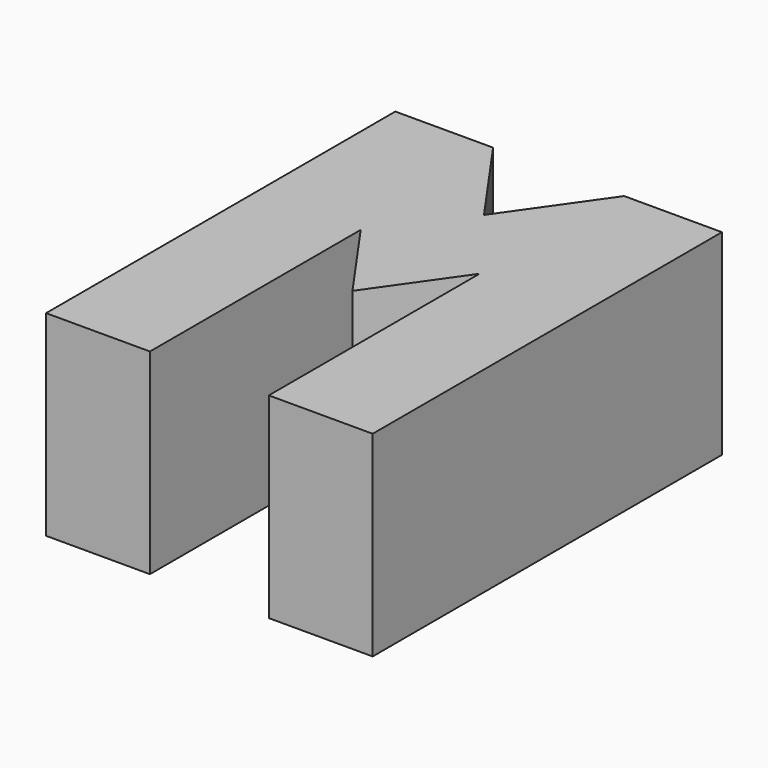
from build123d import *

# Parameters (mm, degrees)
F0_W          = 29.8302113987
F0_H          = 9.2097856104
F1_DEPTH      = 25.4
F2_T1_DEPTH   = 25.4
F2_T3_DEPTH   = 15.24
F2_T5_DEPTH   = 56.4671399768
F2_T7_DEPTH   = 44.9504289544
F2_T9_DEPTH   = 56.4670330548
F2_T11_DEPTH  = 20.32
F2_T13_DEPTH  = 20.3101045111
F2_T15_DEPTH  = 50.8
F2_T20_DEPTH  = 5.08
F2_T26_DEPTH  = 5.08
F2_T32_DEPTH  = 5.08
F2_T38_DEPTH  = 5.08
F2_S43_W      = 5.08
F2_S43_H      = 5.08
F2_T44_DEPTH  = 5.08
F2_S49_W      = 5.08
F2_S49_H      = 5.08
F2_T50_DEPTH  = 5.08
F2_S55_W      = 5.08
F2_S55_H      = 5.08
F2_T56_DEPTH  = 5.08
F2_S61_W      = 5.08
F2_S61_H      = 5.08
F2_T62_DEPTH  = 5.08
F2_T65_DEPTH  = 11.1376243347
F2_T67_DEPTH  = 11.5693333262
F2_T69_DEPTH  = 19.6702113987
F2_S73_W      = 5.08
F2_S73_H      = 5.08
F2_T74_DEPTH  = 5.08
F2_S79_W      = 5.08
F2_S79_H      = 5.08
F2_T80_DEPTH  = 5.08
F2_S85_W      = 5.08
F2_S85_H      = 5.08
F2_T86_DEPTH  = 5.08
F2_S91_W      = 5.08
F2_S91_H      = 5.08
F2_T92_DEPTH  = 5.08
F2_T96_ANGLE  = 90
F2_T98_ANGLE  = 90
F2_T100_ANGLE = 90
F2_T102_ANGLE = 90
F2_T104_ANGLE = 90
F2_T106_ANGLE = 90
F2_T108_ANGLE = 90
F2_T110_ANGLE = 90
F2_T112_ANGLE = 90
F2_T114_ANGLE = 90
F2_T116_ANGLE = 90
F2_T118_ANGLE = 90
F3_DEPTH      = 25.4
F6_DEPTH      = 25.4


# Not quite as in the source:
# - a fillet or chamfer that OpenCascade refuses, or shapes differently, is made with other operations: its cross-section is extruded or revolved along the edge and cut away or added


with BuildPart() as f1:
    # F0 (on Top) → F1 (new body)
    with BuildSketch(Plane.XY):
        Polygon((-27.6151056993, 52.1290511863), (-27.6151056993, 0), (-14.9151056993, 0), (-14.9151056993, 21.7293333262), (-14.9151056993, 30.9391189367), (-14.9151056993, 52.2367432714), (14.9151056993, 52.2367432714), (14.9151056993, 30.9391189367), (14.9151056993, 21.7293333262), (14.9151056993, 0), (27.6151056993, 0), (27.4854470044, 66.6270330548), (-27.6151056993, 66.6270330548), align=None)
        with Locations((0, 26.3342261314)):
            Rectangle(F0_W, F0_H)
    extrude(amount=F1_DEPTH)

    # F2: fillet of radius 5.08 on 36 edges, made by hand

    # F2_s2 → F2_t1 (join)
    with BuildSketch(Plane.XY):
        with BuildLine():
            ThreePointArc((-14.9151056993, 36.0191189367), (-13.4272081478, 32.4270164882), (-9.8351056993, 30.9391189367))
            Line((-9.8351056993, 30.9391189367), (-14.9151056993, 30.9391189367))
            Line((-14.9151056993, 30.9391189367), (-14.9151056993, 36.0191189367))
        make_face()
        with BuildLine():
            ThreePointArc((-14.9151056993, 47.1567432714), (-13.4272081478, 50.7488457198), (-9.8351056993, 52.2367432714))
            Line((-9.8351056993, 52.2367432714), (-14.9151056993, 52.2367432714))
            Line((-14.9151056993, 52.2367432714), (-14.9151056993, 47.1567432714))
        make_face()
        with BuildLine():
            ThreePointArc((9.8351056993, 52.2367432714), (13.4272081478, 50.7488457198), (14.9151056993, 47.1567432714))
            Line((14.9151056993, 47.1567432714), (14.9151056993, 52.2367432714))
            Line((14.9151056993, 52.2367432714), (9.8351056993, 52.2367432714))
        make_face()
        with BuildLine():
            ThreePointArc((14.9151056993, 36.0191189367), (13.4272081478, 32.4270164882), (9.8351056993, 30.9391189367))
            Line((9.8351056993, 30.9391189367), (14.9151056993, 30.9391189367))
            Line((14.9151056993, 30.9391189367), (14.9151056993, 36.0191189367))
        make_face()
        with BuildLine():
            ThreePointArc((9.8351056993, 21.7293333262), (13.4272081478, 20.2414357746), (14.9151056993, 16.6493333262))
            Line((14.9151056993, 16.6493333262), (14.9151056993, 21.7293333262))
            Line((14.9151056993, 21.7293333262), (9.8351056993, 21.7293333262))
        make_face()
        with BuildLine():
            ThreePointArc((-14.9151056993, 16.6493333262), (-13.4272081478, 20.2414357746), (-9.8351056993, 21.7293333262))
            Line((-9.8351056993, 21.7293333262), (-14.9151056993, 21.7293333262))
            Line((-14.9151056993, 21.7293333262), (-14.9151056993, 16.6493333262))
        make_face()
    extrude(amount=F2_T1_DEPTH)

    # F2_s4 → F2_t3 (cut)
    with BuildSketch(Plane.XY.offset(5.08)):
        with BuildLine():
            ThreePointArc((27.6052005914, 5.089885851), (26.1208061363, 1.4913944298), (22.5252102105, 0))
            Line((22.5252102105, 0), (27.6151056993, 0))
            Line((27.6151056993, 0), (27.6052005914, 5.089885851))
        make_face()
        with BuildLine():
            ThreePointArc((22.4153232551, 66.6270330548), (26.0039288252, 65.1426289806), (27.4953136359, 61.5569189059))
            Line((27.4953136359, 61.5569189059), (27.4854470044, 66.6270330548))
            Line((27.4854470044, 66.6270330548), (22.4153232551, 66.6270330548))
        make_face()
        with BuildLine():
            ThreePointArc((-22.5351056993, 66.6270330548), (-26.1272081478, 65.1391355033), (-27.6151056993, 61.5470330548))
            Line((-27.6151056993, 61.5470330548), (-27.6151056993, 66.6270330548))
            Line((-27.6151056993, 66.6270330548), (-22.5351056993, 66.6270330548))
        make_face()
        with BuildLine():
            ThreePointArc((-27.6151056993, 5.08), (-26.1272081478, 1.4878975516), (-22.5351056993, 0))
            Line((-22.5351056993, 0), (-27.6151056993, 0))
            Line((-27.6151056993, 0), (-27.6151056993, 5.08))
        make_face()
    extrude(amount=F2_T3_DEPTH, mode=Mode.SUBTRACT)

    # F2_s6 → F2_t5 (cut)
    with BuildSketch(Plane(origin=(-0.0098005283, 5.0361460274, 0), x_dir=(0, 0, 1), z_dir=(-0.0019460337, 0.9999981065, 0))):
        with BuildLine():
            ThreePointArc((5.08, 27.6150534094), (1.4878975516, 26.1271558579), (0, 22.5350534094))
            Line((0, 22.5350534094), (0, 27.6150534094))
            Line((0, 27.6150534094), (5.08, 27.6150534094))
        make_face()
        with BuildLine():
            ThreePointArc((20.32, 27.6150534094), (23.9121024484, 26.1271558579), (25.4, 22.5350534094))
            Line((25.4, 22.5350534094), (25.4, 27.6150534094))
            Line((25.4, 27.6150534094), (20.32, 27.6150534094))
        make_face()
    extrude(amount=F2_T5_DEPTH, mode=Mode.SUBTRACT)

    # F2_s8 → F2_t7 (cut)
    with BuildSketch(Plane.YZ.offset(-22.5351056993)):
        with BuildLine():
            ThreePointArc((66.6270330548, 5.08), (65.1391355033, 1.4878975516), (61.5470330548, 0))
            Line((61.5470330548, 0), (66.6270330548, 0))
            Line((66.6270330548, 0), (66.6270330548, 5.08))
        make_face()
        with BuildLine():
            ThreePointArc((66.6270330548, 20.32), (65.1391355033, 23.9121024484), (61.5470330548, 25.4))
            Line((61.5470330548, 25.4), (66.6270330548, 25.4))
            Line((66.6270330548, 25.4), (66.6270330548, 20.32))
        make_face()
    extrude(amount=F2_T7_DEPTH, mode=Mode.SUBTRACT)

    # F2_s10 → F2_t9 (cut)
    with BuildSketch(Plane.XZ.offset(-61.5470330548)):
        with BuildLine():
            ThreePointArc((-27.6151056993, 20.32), (-26.1272081478, 23.9121024484), (-22.5351056993, 25.4))
            Line((-22.5351056993, 25.4), (-27.6151056993, 25.4))
            Line((-27.6151056993, 25.4), (-27.6151056993, 20.32))
        make_face()
        with BuildLine():
            ThreePointArc((-27.6151056993, 5.08), (-26.1272081478, 1.4878975516), (-22.5351056993, 0))
            Line((-22.5351056993, 0), (-27.6151056993, 0))
            Line((-27.6151056993, 0), (-27.6151056993, 5.08))
        make_face()
    extrude(amount=F2_T9_DEPTH, mode=Mode.SUBTRACT)

    # F2_s12 → F2_t11 (cut)
    with BuildSketch(Plane.YZ.offset(-22.5351056993)):
        with BuildLine():
            ThreePointArc((5.08, 25.4), (1.4878975516, 23.9121024484), (0, 20.32))
            Line((0, 20.32), (0, 25.4))
            Line((0, 25.4), (5.08, 25.4))
        make_face()
        with BuildLine():
            ThreePointArc((5.08, 0), (1.4878975516, 1.4878975516), (0, 5.08))
            Line((0, 5.08), (0, 0))
            Line((0, 0), (5.08, 0))
        make_face()
    extrude(amount=F2_T11_DEPTH, mode=Mode.SUBTRACT)

    # F2_s14 → F2_t13 (cut)
    with BuildSketch(Plane.YZ.offset(2.2151056993)):
        with BuildLine():
            ThreePointArc((5.08, 25.4), (1.4878975516, 23.9121024484), (0, 20.32))
            Line((0, 20.32), (0, 25.4))
            Line((0, 25.4), (5.08, 25.4))
        make_face()
        with BuildLine():
            ThreePointArc((5.08, 0), (1.4878975516, 1.4878975516), (0, 5.08))
            Line((0, 5.08), (0, 0))
            Line((0, 0), (5.08, 0))
        make_face()
    extrude(amount=F2_T13_DEPTH, mode=Mode.SUBTRACT)

    # F2_s16 → F2_t15 (cut)
    with BuildSketch(Plane.XY.offset(-12.7)):
        with BuildLine():
            ThreePointArc((19.9951056993, 0), (16.4030032509, 1.4878975516), (14.9151056993, 5.08))
            Line((14.9151056993, 5.08), (14.9151056993, 0))
            Line((14.9151056993, 0), (19.9951056993, 0))
        make_face()
        with BuildLine():
            ThreePointArc((-19.9951056993, 0), (-16.4030032509, 1.4878975516), (-14.9151056993, 5.08))
            Line((-14.9151056993, 5.08), (-14.9151056993, 0))
            Line((-14.9151056993, 0), (-19.9951056993, 0))
        make_face()
    extrude(amount=F2_T15_DEPTH, mode=Mode.SUBTRACT)


with BuildPart() as f2_tool18:
    # F2_s19 → F2_t20 (new body)
    with BuildSketch(Plane.XY.offset(5.08)):
        Polygon((22.5252102105, 5.08), (22.5252102105, 0), (27.6151056993, 0), (27.6052005914, 5.089885851), align=None)
    extrude(amount=-F2_T20_DEPTH)

    # F2_s21 → F2_t22 (revolve, cut)
    with BuildSketch(Plane(origin=(22.5252102105, 5.08, 5.08), x_dir=(-0.7077944736, 0.7064184193, 0), z_dir=(-0.7064184193, -0.7077944736, 0))):
        with BuildLine():
            ThreePointArc((0, -5.08), (5.08, 0), (0, 5.08))
            Line((0, 5.08), (0, -5.08))
        make_face()
    revolve(axis=Axis((22.5252102105, 5.08, 5.08), (0, 0, -1)), mode=Mode.SUBTRACT)


with BuildPart() as f1_1:
    add(f1.part)

    # F2_t17: cut F2_tool18
    add(f2_tool18.part, mode=Mode.SUBTRACT)


with BuildPart() as f2_tool24:
    # F2_s25 → F2_t26 (new body)
    with BuildSketch(Plane.XY.offset(20.32)):
        Polygon((22.5252102105, 5.08), (22.5252102105, 0), (27.6151056993, 0), (27.6052005914, 5.089885851), align=None)
    extrude(amount=F2_T26_DEPTH)

    # F2_s27 → F2_t28 (revolve, cut)
    with BuildSketch(Plane(origin=(22.5252102105, 5.08, 20.32), x_dir=(-0.7077944736, 0.7064184193, 0), z_dir=(0.7064184193, 0.7077944736, 0))):
        with BuildLine():
            ThreePointArc((0, -5.08), (5.08, 0), (0, 5.08))
            Line((0, 5.08), (0, -5.08))
        make_face()
    revolve(axis=Axis((22.5252102105, 5.08, 20.32), (0, 0, 1)), mode=Mode.SUBTRACT)


with BuildPart() as f1_2:
    add(f1_1.part)

    # F2_t23: cut F2_tool24
    add(f2_tool24.part, mode=Mode.SUBTRACT)


with BuildPart() as f2_tool30:
    # F2_s31 → F2_t32 (new body)
    with BuildSketch(Plane.XY.offset(5.08)):
        Polygon((22.4153232551, 61.5470330548), (22.4153232551, 66.6270330548), (27.4854470044, 66.6270330548), (27.4953136359, 61.5569189059), align=None)
    extrude(amount=-F2_T32_DEPTH)

    # F2_s33 → F2_t34 (revolve, cut)
    with BuildSketch(Plane(origin=(22.4153232551, 61.5470330548, 5.08), x_dir=(-0.7064184193, -0.7077944736, 0), z_dir=(0.7077944736, -0.7064184193, 0))):
        with BuildLine():
            ThreePointArc((0, -5.08), (5.08, 0), (0, 5.08))
            Line((0, 5.08), (0, -5.08))
        make_face()
    revolve(axis=Axis((22.4153232551, 61.5470330548, 5.08), (0, 0, -1)), mode=Mode.SUBTRACT)


with BuildPart() as f1_3:
    add(f1_2.part)

    # F2_t29: cut F2_tool30
    add(f2_tool30.part, mode=Mode.SUBTRACT)


with BuildPart() as f2_tool36:
    # F2_s37 → F2_t38 (new body)
    with BuildSketch(Plane.XY.offset(20.32)):
        Polygon((22.4153232551, 61.5470330548), (22.4153232551, 66.6270330548), (27.4854470044, 66.6270330548), (27.4953136359, 61.5569189059), align=None)
    extrude(amount=F2_T38_DEPTH)

    # F2_s39 → F2_t40 (revolve, cut)
    with BuildSketch(Plane(origin=(22.4153232551, 61.5470330548, 20.32), x_dir=(-0.7064184193, -0.7077944736, 0), z_dir=(-0.7077944736, 0.7064184193, 0))):
        with BuildLine():
            ThreePointArc((0, -5.08), (5.08, 0), (0, 5.08))
            Line((0, 5.08), (0, -5.08))
        make_face()
    revolve(axis=Axis((22.4153232551, 61.5470330548, 20.32), (0, 0, 1)), mode=Mode.SUBTRACT)


with BuildPart() as f1_4:
    add(f1_3.part)

    # F2_t35: cut F2_tool36
    add(f2_tool36.part, mode=Mode.SUBTRACT)


with BuildPart() as f2_tool42:
    # F2_s43 → F2_t44 (new body)
    with BuildSketch(Plane.XZ.offset(-61.5470330548)):
        with Locations((-25.0751056993, 2.54)):
            Rectangle(F2_S43_W, F2_S43_H)
    extrude(amount=-F2_T44_DEPTH)

    # F2_s45 → F2_t46 (revolve, cut)
    with BuildSketch(Plane(origin=(-22.5351056993, 61.5470330548, 5.08), x_dir=(0.7071067812, 0, 0.7071067812), z_dir=(-0.7071067812, 0, 0.7071067812))):
        with BuildLine():
            ThreePointArc((0, -5.08), (5.08, 0), (0, 5.08))
            Line((0, 5.08), (0, -5.08))
        make_face()
    revolve(axis=Axis((-22.5351056993, 61.5470330548, 5.08), (0, 1, 0)), mode=Mode.SUBTRACT)


with BuildPart() as f1_5:
    add(f1_4.part)

    # F2_t41: cut F2_tool42
    add(f2_tool42.part, mode=Mode.SUBTRACT)


with BuildPart() as f2_tool48:
    # F2_s49 → F2_t50 (new body)
    with BuildSketch(Plane.XZ.offset(-61.5470330548)):
        with Locations((-25.0751056993, 22.86)):
            Rectangle(F2_S49_W, F2_S49_H)
    extrude(amount=-F2_T50_DEPTH)

    # F2_s51 → F2_t52 (revolve, cut)
    with BuildSketch(Plane(origin=(-22.5351056993, 61.5470330548, 20.32), x_dir=(0.7071067812, 0, -0.7071067812), z_dir=(0.7071067812, 0, 0.7071067812))):
        with BuildLine():
            ThreePointArc((0, -5.08), (5.08, 0), (0, 5.08))
            Line((0, 5.08), (0, -5.08))
        make_face()
    revolve(axis=Axis((-22.5351056993, 61.5470330548, 20.32), (0, 1, 0)), mode=Mode.SUBTRACT)


with BuildPart() as f1_6:
    add(f1_5.part)

    # F2_t47: cut F2_tool48
    add(f2_tool48.part, mode=Mode.SUBTRACT)


with BuildPart() as f2_tool54:
    # F2_s55 → F2_t56 (new body)
    with BuildSketch(Plane.YZ.offset(-22.5351056993)):
        with Locations((2.54, 22.86)):
            Rectangle(F2_S55_W, F2_S55_H)
    extrude(amount=-F2_T56_DEPTH)

    # F2_s57 → F2_t58 (revolve, cut)
    with BuildSketch(Plane(origin=(-22.5351056993, 5.08, 20.32), x_dir=(0, 0.7071067812, -0.7071067812), z_dir=(0, 0.7071067812, 0.7071067812))):
        with BuildLine():
            ThreePointArc((0, -5.08), (5.08, 0), (0, 5.08))
            Line((0, 5.08), (0, -5.08))
        make_face()
    revolve(axis=Axis((-22.5351056993, 5.08, 20.32), (-1, 0, 0)), mode=Mode.SUBTRACT)


with BuildPart() as f1_7:
    add(f1_6.part)

    # F2_t53: cut F2_tool54
    add(f2_tool54.part, mode=Mode.SUBTRACT)


with BuildPart() as f2_tool60:
    # F2_s61 → F2_t62 (new body)
    with BuildSketch(Plane.YZ.offset(-22.5351056993)):
        with Locations((2.54, 2.54)):
            Rectangle(F2_S61_W, F2_S61_H)
    extrude(amount=-F2_T62_DEPTH)

    # F2_s63 → F2_t64 (revolve, cut)
    with BuildSketch(Plane(origin=(-22.5351056993, 5.08, 5.08), x_dir=(0, 0.7071067812, 0.7071067812), z_dir=(0, -0.7071067812, 0.7071067812))):
        with BuildLine():
            ThreePointArc((0, -5.08), (5.08, 0), (0, 5.08))
            Line((0, 5.08), (0, -5.08))
        make_face()
    revolve(axis=Axis((-22.5351056993, 5.08, 5.08), (-1, 0, 0)), mode=Mode.SUBTRACT)


with BuildPart() as f1_8:
    add(f1_7.part)

    # F2_t59: cut F2_tool60
    add(f2_tool60.part, mode=Mode.SUBTRACT)

    # F2_s66 → F2_t65 (cut)
    with BuildSketch(Plane.XZ.offset(-47.1567432714)):
        with BuildLine():
            ThreePointArc((-19.9951056993, 0), (-16.4030032509, 1.4878975516), (-14.9151056993, 5.08))
            Line((-14.9151056993, 5.08), (-14.9151056993, 0))
            Line((-14.9151056993, 0), (-19.9951056993, 0))
        make_face()
        with BuildLine():
            ThreePointArc((-19.9951056993, 25.4), (-16.4030032509, 23.9121024484), (-14.9151056993, 20.32))
            Line((-14.9151056993, 20.32), (-14.9151056993, 25.4))
            Line((-14.9151056993, 25.4), (-19.9951056993, 25.4))
        make_face()
        with BuildLine():
            ThreePointArc((19.9951056993, 25.4), (16.4030032509, 23.9121024484), (14.9151056993, 20.32))
            Line((14.9151056993, 20.32), (14.9151056993, 25.4))
            Line((14.9151056993, 25.4), (19.9951056993, 25.4))
        make_face()
        with BuildLine():
            ThreePointArc((19.9951056993, 0), (16.4030032509, 1.4878975516), (14.9151056993, 5.08))
            Line((14.9151056993, 5.08), (14.9151056993, 0))
            Line((14.9151056993, 0), (19.9951056993, 0))
        make_face()
    extrude(amount=F2_T65_DEPTH, mode=Mode.SUBTRACT)

    # F2_s68 → F2_t67 (cut)
    with BuildSketch(Plane.XZ.offset(-16.6493333262)):
        with BuildLine():
            ThreePointArc((-19.9951056993, 25.4), (-16.4030032509, 23.9121024484), (-14.9151056993, 20.32))
            Line((-14.9151056993, 20.32), (-14.9151056993, 25.4))
            Line((-14.9151056993, 25.4), (-19.9951056993, 25.4))
        make_face()
        with BuildLine():
            ThreePointArc((19.9951056993, 25.4), (16.4030032509, 23.9121024484), (14.9151056993, 20.32))
            Line((14.9151056993, 20.32), (14.9151056993, 25.4))
            Line((14.9151056993, 25.4), (19.9951056993, 25.4))
        make_face()
        with BuildLine():
            ThreePointArc((19.9951056993, 0), (16.4030032509, 1.4878975516), (14.9151056993, 5.08))
            Line((14.9151056993, 5.08), (14.9151056993, 0))
            Line((14.9151056993, 0), (19.9951056993, 0))
        make_face()
        with BuildLine():
            ThreePointArc((-19.9951056993, 0), (-16.4030032509, 1.4878975516), (-14.9151056993, 5.08))
            Line((-14.9151056993, 5.08), (-14.9151056993, 0))
            Line((-14.9151056993, 0), (-19.9951056993, 0))
        make_face()
    extrude(amount=F2_T67_DEPTH, mode=Mode.SUBTRACT)

    # F2_s70 → F2_t69 (cut)
    with BuildSketch(Plane.YZ.offset(-9.8351056993)):
        with BuildLine():
            ThreePointArc((26.8093333262, 25.4), (23.2172308778, 23.9121024484), (21.7293333262, 20.32))
            Line((21.7293333262, 20.32), (21.7293333262, 25.4))
            Line((21.7293333262, 25.4), (26.8093333262, 25.4))
        make_face()
        with BuildLine():
            ThreePointArc((57.3167432714, 25.4), (53.7246408229, 23.9121024484), (52.2367432714, 20.32))
            Line((52.2367432714, 20.32), (52.2367432714, 25.4))
            Line((52.2367432714, 25.4), (57.3167432714, 25.4))
        make_face()
        with BuildLine():
            ThreePointArc((25.8591189367, 25.4), (29.4512213851, 23.9121024484), (30.9391189367, 20.32))
            Line((30.9391189367, 20.32), (30.9391189367, 25.4))
            Line((30.9391189367, 25.4), (25.8591189367, 25.4))
        make_face()
        with BuildLine():
            ThreePointArc((26.8093333262, 0), (23.2172308778, 1.4878975516), (21.7293333262, 5.08))
            Line((21.7293333262, 5.08), (21.7293333262, 0))
            Line((21.7293333262, 0), (26.8093333262, 0))
        make_face()
        with BuildLine():
            ThreePointArc((57.3167432714, 0), (53.7246408229, 1.4878975516), (52.2367432714, 5.08))
            Line((52.2367432714, 5.08), (52.2367432714, 0))
            Line((52.2367432714, 0), (57.3167432714, 0))
        make_face()
        with BuildLine():
            ThreePointArc((25.8591189367, 0), (29.4512213851, 1.4878975516), (30.9391189367, 5.08))
            Line((30.9391189367, 5.08), (30.9391189367, 0))
            Line((30.9391189367, 0), (25.8591189367, 0))
        make_face()
    extrude(amount=F2_T69_DEPTH, mode=Mode.SUBTRACT)


with BuildPart() as f2_tool72:
    # F2_s73 → F2_t74 (new body)
    with BuildSketch(Plane.XY.offset(5.08)):
        with Locations((-17.4551056993, 2.54)):
            Rectangle(F2_S73_W, F2_S73_H)
    extrude(amount=-F2_T74_DEPTH)

    # F2_s75 → F2_t76 (revolve, cut)
    with BuildSketch(Plane(origin=(-19.9951056993, 5.08, 5.08), x_dir=(-0.7071067812, 0.7071067812, 0), z_dir=(-0.7071067812, -0.7071067812, 0))):
        with BuildLine():
            ThreePointArc((0, -5.08), (5.08, 0), (0, 5.08))
            Line((0, 5.08), (0, -5.08))
        make_face()
    revolve(axis=Axis((-19.9951056993, 5.08, 5.08), (0, 0, -1)), mode=Mode.SUBTRACT)


with BuildPart() as f1_9:
    add(f1_8.part)

    # F2_t71: cut F2_tool72
    add(f2_tool72.part, mode=Mode.SUBTRACT)


with BuildPart() as f2_tool78:
    # F2_s79 → F2_t80 (new body)
    with BuildSketch(Plane.XY.offset(5.08)):
        with Locations((17.4551056993, 2.54)):
            Rectangle(F2_S79_W, F2_S79_H)
    extrude(amount=-F2_T80_DEPTH)

    # F2_s81 → F2_t82 (revolve, cut)
    with BuildSketch(Plane(origin=(19.9951056993, 5.08, 5.08), x_dir=(0.7071067812, 0.7071067812, 0), z_dir=(-0.7071067812, 0.7071067812, 0))):
        with BuildLine():
            ThreePointArc((0, -5.08), (5.08, 0), (0, 5.08))
            Line((0, 5.08), (0, -5.08))
        make_face()
    revolve(axis=Axis((19.9951056993, 5.08, 5.08), (0, 0, -1)), mode=Mode.SUBTRACT)


with BuildPart() as f1_10:
    add(f1_9.part)

    # F2_t77: cut F2_tool78
    add(f2_tool78.part, mode=Mode.SUBTRACT)


with BuildPart() as f2_tool84:
    # F2_s85 → F2_t86 (new body)
    with BuildSketch(Plane.XY.offset(20.32)):
        with Locations((17.4551056993, 2.54)):
            Rectangle(F2_S85_W, F2_S85_H)
    extrude(amount=F2_T86_DEPTH)

    # F2_s87 → F2_t88 (revolve, cut)
    with BuildSketch(Plane(origin=(19.9951056993, 5.08, 20.32), x_dir=(0.7071067812, 0.7071067812, 0), z_dir=(0.7071067812, -0.7071067812, 0))):
        with BuildLine():
            ThreePointArc((0, -5.08), (5.08, 0), (0, 5.08))
            Line((0, 5.08), (0, -5.08))
        make_face()
    revolve(axis=Axis((19.9951056993, 5.08, 20.32), (0, 0, 1)), mode=Mode.SUBTRACT)


with BuildPart() as f1_11:
    add(f1_10.part)

    # F2_t83: cut F2_tool84
    add(f2_tool84.part, mode=Mode.SUBTRACT)


with BuildPart() as f2_tool90:
    # F2_s91 → F2_t92 (new body)
    with BuildSketch(Plane.XY.offset(20.32)):
        with Locations((-17.4551056993, 2.54)):
            Rectangle(F2_S91_W, F2_S91_H)
    extrude(amount=F2_T92_DEPTH)

    # F2_s93 → F2_t94 (revolve, cut)
    with BuildSketch(Plane(origin=(-19.9951056993, 5.08, 20.32), x_dir=(-0.7071067812, 0.7071067812, 0), z_dir=(0.7071067812, 0.7071067812, 0))):
        with BuildLine():
            ThreePointArc((0, -5.08), (5.08, 0), (0, 5.08))
            Line((0, 5.08), (0, -5.08))
        make_face()
    revolve(axis=Axis((-19.9951056993, 5.08, 20.32), (0, 0, 1)), mode=Mode.SUBTRACT)


with BuildPart() as f1_12:
    add(f1_11.part)

    # F2_t89: cut F2_tool90
    add(f2_tool90.part, mode=Mode.SUBTRACT)

    # F2_s95 → F2_t96 (revolve, cut)
    with BuildSketch(Plane.XZ.offset(-36.0191189367)):
        with BuildLine():
            ThreePointArc((19.9951056993, 0), (16.4030032509, 1.4878975516), (14.9151056993, 5.08))
            Line((14.9151056993, 5.08), (14.9151056993, 0))
            Line((14.9151056993, 0), (19.9951056993, 0))
        make_face()
    revolve(axis=Axis((9.8351056993, 36.0191189367, 0), (0, 0, -1)), revolution_arc=F2_T96_ANGLE, mode=Mode.SUBTRACT)

    # F2_s97 → F2_t98 (revolve, cut)
    with BuildSketch(Plane.XZ.offset(-36.0191189367)):
        with BuildLine():
            ThreePointArc((-19.9951056993, 0), (-16.4030032509, 1.4878975516), (-14.9151056993, 5.08))
            Line((-14.9151056993, 5.08), (-14.9151056993, 0))
            Line((-14.9151056993, 0), (-19.9951056993, 0))
        make_face()
    revolve(axis=Axis((-9.8351056993, 36.0191189367, 0), (0, 0, 1)), revolution_arc=F2_T98_ANGLE, mode=Mode.SUBTRACT)

    # F2_s99 → F2_t100 (revolve, cut)
    with BuildSketch(Plane.XZ.offset(-47.1567432714)):
        with BuildLine():
            ThreePointArc((-19.9951056993, 0), (-16.4030032509, 1.4878975516), (-14.9151056993, 5.08))
            Line((-14.9151056993, 5.08), (-14.9151056993, 0))
            Line((-14.9151056993, 0), (-19.9951056993, 0))
        make_face()
    revolve(axis=Axis((-9.8351056993, 47.1567432714, 0), (0, 0, -1)), revolution_arc=F2_T100_ANGLE, mode=Mode.SUBTRACT)

    # F2_s101 → F2_t102 (revolve, cut)
    with BuildSketch(Plane.YZ.offset(9.8351056993)):
        with BuildLine():
            ThreePointArc((57.3167432714, 0), (53.7246408229, 1.4878975516), (52.2367432714, 5.08))
            Line((52.2367432714, 5.08), (52.2367432714, 0))
            Line((52.2367432714, 0), (57.3167432714, 0))
        make_face()
    revolve(axis=Axis((9.8351056993, 47.1567432714, 0), (0, 0, -1)), revolution_arc=F2_T102_ANGLE, mode=Mode.SUBTRACT)

    # F2_s103 → F2_t104 (revolve, cut)
    with BuildSketch(Plane.XZ.offset(-16.6493333262)):
        with BuildLine():
            ThreePointArc((-19.9951056993, 0), (-16.4030032509, 1.4878975516), (-14.9151056993, 5.08))
            Line((-14.9151056993, 5.08), (-14.9151056993, 0))
            Line((-14.9151056993, 0), (-19.9951056993, 0))
        make_face()
    revolve(axis=Axis((-9.8351056993, 16.6493333262, 0), (0, 0, -1)), revolution_arc=F2_T104_ANGLE, mode=Mode.SUBTRACT)

    # F2_s105 → F2_t106 (revolve, cut)
    with BuildSketch(Plane.YZ.offset(9.8351056993)):
        with BuildLine():
            ThreePointArc((26.8093333262, 0), (23.2172308778, 1.4878975516), (21.7293333262, 5.08))
            Line((21.7293333262, 5.08), (21.7293333262, 0))
            Line((21.7293333262, 0), (26.8093333262, 0))
        make_face()
    revolve(axis=Axis((9.8351056993, 16.6493333262, 0), (0, 0, -1)), revolution_arc=F2_T106_ANGLE, mode=Mode.SUBTRACT)

    # F2_s107 → F2_t108 (revolve, cut)
    with BuildSketch(Plane.XZ.offset(-36.0191189367)):
        with BuildLine():
            ThreePointArc((19.9951056993, 25.4), (16.4030032509, 23.9121024484), (14.9151056993, 20.32))
            Line((14.9151056993, 20.32), (14.9151056993, 25.4))
            Line((14.9151056993, 25.4), (19.9951056993, 25.4))
        make_face()
    revolve(axis=Axis((9.8351056993, 36.0191189367, 25.4), (0, 0, -1)), revolution_arc=F2_T108_ANGLE, mode=Mode.SUBTRACT)

    # F2_s109 → F2_t110 (revolve, cut)
    with BuildSketch(Plane.XZ.offset(-36.0191189367)):
        with BuildLine():
            ThreePointArc((-19.9951056993, 25.4), (-16.4030032509, 23.9121024484), (-14.9151056993, 20.32))
            Line((-14.9151056993, 20.32), (-14.9151056993, 25.4))
            Line((-14.9151056993, 25.4), (-19.9951056993, 25.4))
        make_face()
    revolve(axis=Axis((-9.8351056993, 36.0191189367, 25.4), (0, 0, 1)), revolution_arc=F2_T110_ANGLE, mode=Mode.SUBTRACT)

    # F2_s111 → F2_t112 (revolve, cut)
    with BuildSketch(Plane.YZ.offset(9.8351056993)):
        with BuildLine():
            ThreePointArc((57.3167432714, 25.4), (53.7246408229, 23.9121024484), (52.2367432714, 20.32))
            Line((52.2367432714, 20.32), (52.2367432714, 25.4))
            Line((52.2367432714, 25.4), (57.3167432714, 25.4))
        make_face()
    revolve(axis=Axis((9.8351056993, 47.1567432714, 25.4), (0, 0, -1)), revolution_arc=F2_T112_ANGLE, mode=Mode.SUBTRACT)

    # F2_s113 → F2_t114 (revolve, cut)
    with BuildSketch(Plane.XZ.offset(-47.1567432714)):
        with BuildLine():
            ThreePointArc((-19.9951056993, 25.4), (-16.4030032509, 23.9121024484), (-14.9151056993, 20.32))
            Line((-14.9151056993, 20.32), (-14.9151056993, 25.4))
            Line((-14.9151056993, 25.4), (-19.9951056993, 25.4))
        make_face()
    revolve(axis=Axis((-9.8351056993, 47.1567432714, 25.4), (0, 0, -1)), revolution_arc=F2_T114_ANGLE, mode=Mode.SUBTRACT)

    # F2_s115 → F2_t116 (revolve, cut)
    with BuildSketch(Plane.YZ.offset(9.8351056993)):
        with BuildLine():
            ThreePointArc((26.8093333262, 25.4), (23.2172308778, 23.9121024484), (21.7293333262, 20.32))
            Line((21.7293333262, 20.32), (21.7293333262, 25.4))
            Line((21.7293333262, 25.4), (26.8093333262, 25.4))
        make_face()
    revolve(axis=Axis((9.8351056993, 16.6493333262, 25.4), (0, 0, -1)), revolution_arc=F2_T116_ANGLE, mode=Mode.SUBTRACT)

    # F2_s117 → F2_t118 (revolve, cut)
    with BuildSketch(Plane.XZ.offset(-16.6493333262)):
        with BuildLine():
            ThreePointArc((-19.9951056993, 25.4), (-16.4030032509, 23.9121024484), (-14.9151056993, 20.32))
            Line((-14.9151056993, 20.32), (-14.9151056993, 25.4))
            Line((-14.9151056993, 25.4), (-19.9951056993, 25.4))
        make_face()
    revolve(axis=Axis((-9.8351056993, 16.6493333262, 25.4), (0, 0, -1)), revolution_arc=F2_T118_ANGLE, mode=Mode.SUBTRACT)

    # F3 (add): a face of the model
    f3_faces = [f1_12.faces().sort_by_distance(p)[0] for p in [
        (0, 58.0391668239, 25.4),
    ]]
    extrude(f3_faces, amount=F3_DEPTH)


with BuildPart() as f6:
    # F5 (on Top) → F6 (new body)
    with BuildSketch(Plane.XY):
        Polygon((-8.4902700037, 56.5538331866), (-21.153723821, 56.5538331866), (-21.153723821, 0), (-7.6992294526, 0), (-7.6992294526, 34.1299795523), (0, 23.1683626771), (0, 44.4659888744), align=None)
        Polygon((8.4902700037, 56.5538331866), (0, 44.4659888744), (0, 23.1683626771), (7.6992294526, 34.1299795523), (7.6992294526, 0), (21.153723821, 0), (21.153723821, 56.5538331866), align=None)
    extrude(amount=F6_DEPTH)


solid = f6.part
